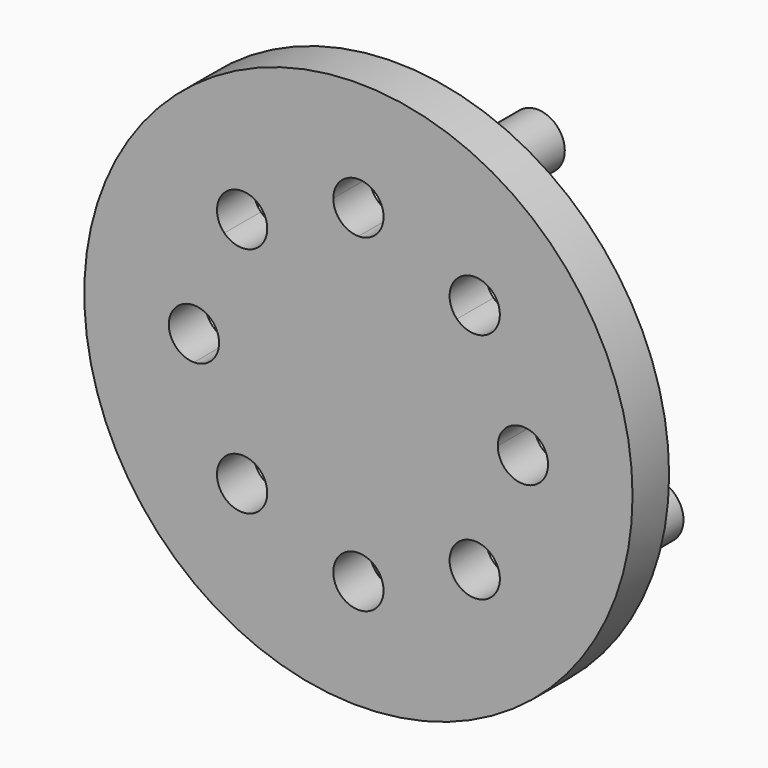
from build123d import *

# Parameters (mm, degrees)
F0_R            = 30
F1_DEPTH        = 5
F3_DEPTH        = 25
F3_COPIES_COUNT = 8
F5_DEPTH        = 8
F5_COPIES_COUNT = 4


# Not quite as in the source:
# - a pattern or mirror of a feature is missing from the dataset's text; its kind, count and spacing are read off the source's solid
# - a feature names something its author has since deleted; it is built from what else it names


with BuildPart() as f1:
    # F0 (on Front) → F1 (new body)
    with BuildSketch(Plane.XZ):
        Circle(F0_R)
    extrude(amount=F1_DEPTH)

    # F2 (on face) → F3 (cut)
    with BuildSketch(Plane.XZ.offset(5)):
        with BuildLine():
            ThreePointArc((0, -15.25), (-1.9445436483, -19.9445436483), (2.75, -18))
            ThreePointArc((2.75, -18), (1.9445436483, -16.0554563517), (0, -15.25))
        make_face()
    f3 = extrude(amount=-F3_DEPTH, mode=Mode.SUBTRACT)

    # F3_copies: F3 ×8 about axis
    f3_copies_axis = Axis((0, 0, 0), (0, 1, 0))
    for i in range(1, F3_COPIES_COUNT):
        add(f3.rotate(f3_copies_axis, i * 360 / F3_COPIES_COUNT), mode=Mode.SUBTRACT)

    # F4 (on face) → F5 (join)
    with BuildSketch(Plane(origin=(0, 0, 0), x_dir=(-1, 0, 0), z_dir=(0, 1, 0))):
        with BuildLine():
            ThreePointArc((-8.0363520797, 19.4014701827), (-6.6899935399, 20.5063980812), (-6.1844023768, 22.1731087803))
            ThreePointArc((-6.1844023768, 22.1731087803), (-11.6788112137, 23.8398194793), (-8.0363520797, 19.4014701827))
        make_face()
    f5 = extrude(amount=F5_DEPTH)

    # F5_copies: F5 ×4 about axis
    f5_copies_axis = Axis((0, 0, 0), (0, 1, 0))
    for i in range(1, F5_COPIES_COUNT):
        add(f5.rotate(f5_copies_axis, i * 360 / F5_COPIES_COUNT))


solid = f1.part
